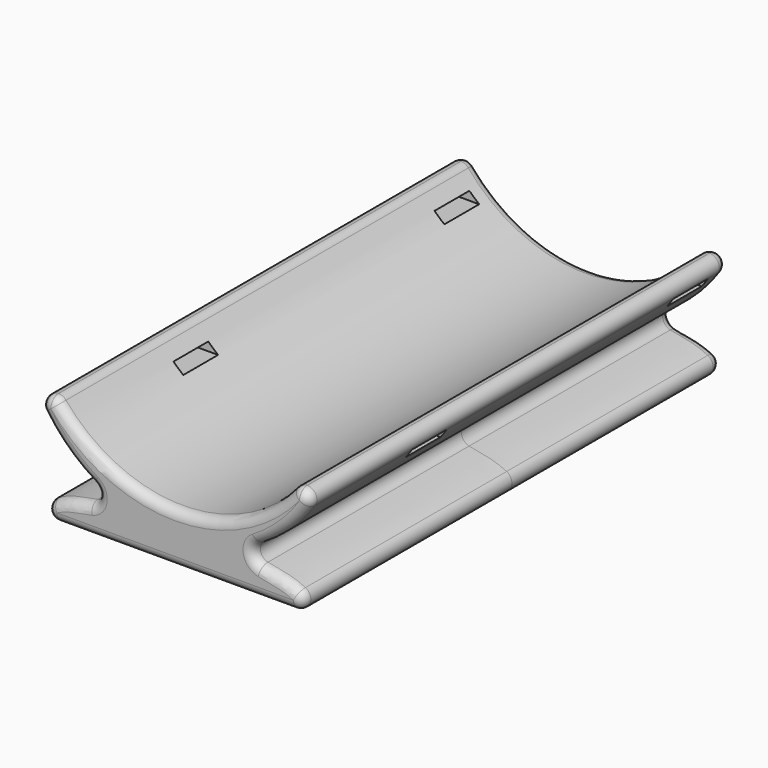
from build123d import *

# Parameters (mm, degrees)
F1_DEPTH      = 60
F1_DEPTH_BACK = 60
F2_R          = 2.22
F3_W          = 10
F3_H          = 2
F4_DEPTH      = 30.8111762664
F4_DEPTH_BACK = 30.8111762664
F5_TEXT_SIZE  = 11.0583153348
F6_DEPTH      = 0.4


# Not quite as in the source:
# - a feature names something its author has since deleted; it is built from what else it names
# - Text() gives the source's letters only with a copy of the font that has no kerning and outlines rounded to 1/6400 em; it was checked with that copy


with BuildPart() as f1:
    # F0 (on Front) → F1 (new body, two sides)
    with BuildSketch(Plane.XZ) as f1_sk:
        with BuildLine():
            add(Edge.make_bspline(
                [(-32.5, 0), (-31.1984516336, 2.9934663266), (-24.662755661, 6.3886345513), (-17.1366381972, 6.461150832), (-15.1692357036, 8.6456461155)],
                knots=[0, 0, 0, 0, 0.5012569461, 1, 1, 1, 1], degree=3))
            Line((-32.5, 0), (32.5, 0))
            add(Edge.make_bspline(
                [(32.5, 0), (31.1984516336, 2.9934663266), (24.662755661, 6.3886345513), (17.1366381972, 6.461150832), (15.1692357036, 8.6456461155)],
                knots=[0, 0, 0, 0, 0.5012569461, 1, 1, 1, 1], degree=3))
            ThreePointArc((15.1692357036, 8.6456461155), (0, 5.3654417235), (-15.1692357036, 8.6456461155))
        make_face()
        with BuildLine():
            Line((15.1692357036, 8.6456461155), (-15.1692357036, 8.6456461155))
            ThreePointArc((-15.1692357036, 8.6456461155), (0, 5.3654417235), (15.1692357036, 8.6456461155))
        make_face()
        with BuildLine():
            ThreePointArc((-32.5, 25), (-25.198318017, 15.3777053661), (-15.1692357036, 8.6456461155))
            Line((-15.1692357036, 8.6456461155), (15.1692357036, 8.6456461155))
            ThreePointArc((15.1692357036, 8.6456461155), (25.198318017, 15.3777053661), (32.5, 25))
            Line((32.5, 25), (27.5, 25))
            ThreePointArc((27.5, 25), (0, 11.6506350946), (-27.5, 25))
            Line((-27.5, 25), (-32.5, 25))
        make_face()
    extrude(amount=F1_DEPTH)
    extrude(f1_sk.sketch, amount=-F1_DEPTH_BACK)

    # F2
    f2_edges = [f1.edges().sort_by_distance(p)[0] for p in [
        (30, -60, 25),
        (-30, -60, 25),
        (0, -60, 11.650635),
        (0, -60, 0),
        (-27.5, 0, 25),
        (0, 60, 11.650635),
        (30, 60, 25),
        (-30, 60, 25),
        (0, 60, 0),
        (27.5, 0, 25),
        (25.198318, 60, 15.377705),
        (32.5, 0, 25),
        (24.538862, 60, 5.527065),
        (-25.198318, 60, 15.377705),
        (-24.538862, 60, 5.527065),
        (-25.198318, -60, 15.377705),
        (-24.538862, -60, 5.527065),
        (24.538862, -60, 5.527065),
        (25.198318, -60, 15.377705),
        (15.169236, -30, 8.645646),
        (15.169236, 30, 8.645646),
        (-15.169236, -30, 8.645646),
        (-15.169236, 30, 8.645646),
        (-32.5, -30, 0),
        (32.5, -30, 0),
        (32.5, 30, 0),
        (-32.5, 0, 25),
        (-32.5, 30, 0),
    ]]
    fillet(f2_edges, radius=F2_R)

    # F3 (on Right) → F4 (cut, two sides)
    with BuildSketch(Plane.YZ) as f4_sk:
        with Locations((50, 20.537878324)):
            Rectangle(F3_W, F3_H)
        with Locations((-25, 20.537878324)):
            Rectangle(F3_W, F3_H)
    extrude(amount=F4_DEPTH, mode=Mode.SUBTRACT)
    extrude(f4_sk.sketch, amount=-F4_DEPTH_BACK, mode=Mode.SUBTRACT)

    # F5 (on face) → F6 (cut)
    with BuildSketch(Plane(origin=(0, 0, 0), x_dir=(1, 0, 0), z_dir=(0, 0, -1))):
        with Locations(Location((-3.9809935205, 50), (0, 0, -90))):
            Text('Thorsten Waßmuth', F5_TEXT_SIZE, font='Open Sans', text_align=(TextAlign.LEFT, TextAlign.BOTTOM))
    extrude(amount=-F6_DEPTH, mode=Mode.SUBTRACT)


solid = f1.part
